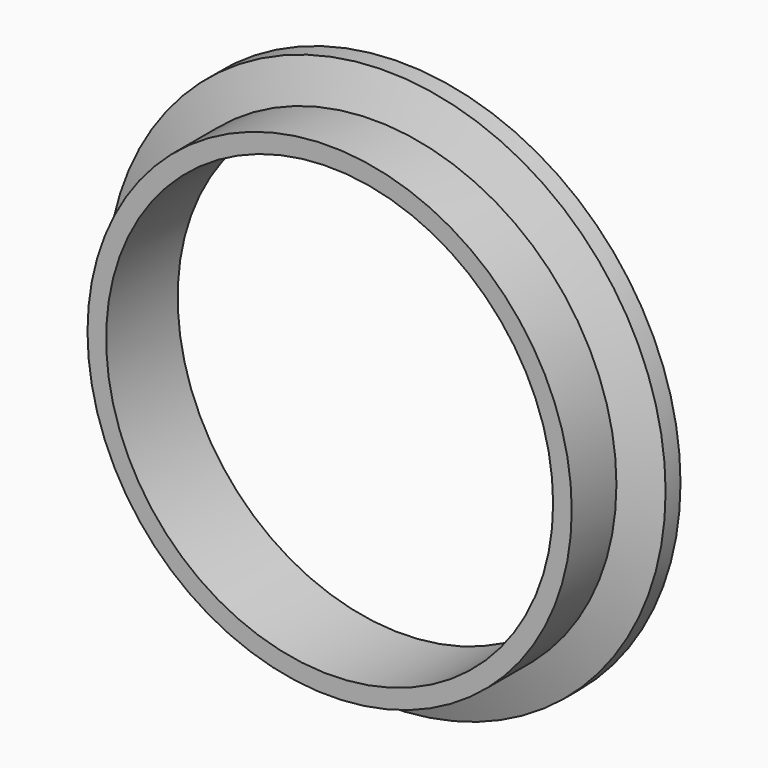
from build123d import *

# Parameters (mm, degrees)
F0_R     = 47.625
F0_R_2   = 38.1
F1_DEPTH = 15.24
F2_R     = 47.625
F2_R_2   = 41.275
F3_DEPTH = 12.065
F4_SIZE2 = 6.34999
F4_SIZE  = 2.53999


# Not quite as in the source:
# - a fillet or chamfer is up to 0.001 mm smaller than in the source, because OpenCascade refuses the exact size


with BuildPart() as f1:
    # F0 (on Front) → F1 (new body)
    with BuildSketch(Plane.XZ):
        Circle(F0_R)
        Circle(F0_R_2, mode=Mode.SUBTRACT)
    extrude(amount=F1_DEPTH)

    # F2 (on face) → F3 (cut)
    with BuildSketch(Plane.XZ.offset(15.24)):
        Circle(F2_R)
        Circle(F2_R_2, mode=Mode.SUBTRACT)
    extrude(amount=-F3_DEPTH, mode=Mode.SUBTRACT)

    # F4 (size 2.54 and 6.35 in the source; OpenCascade refuses exactly that, so slightly less here)
    f4_edges = [f1.edges().sort_by_distance(p)[0] for p in [
        (-41.275, -3.175, 0),
    ]]
    f4_side = f1.faces().sort_by_distance((-41.275, -9.2075, 0))[0]
    chamfer(f4_edges, length=F4_SIZE, length2=F4_SIZE2, reference=f4_side)


solid = f1.part
